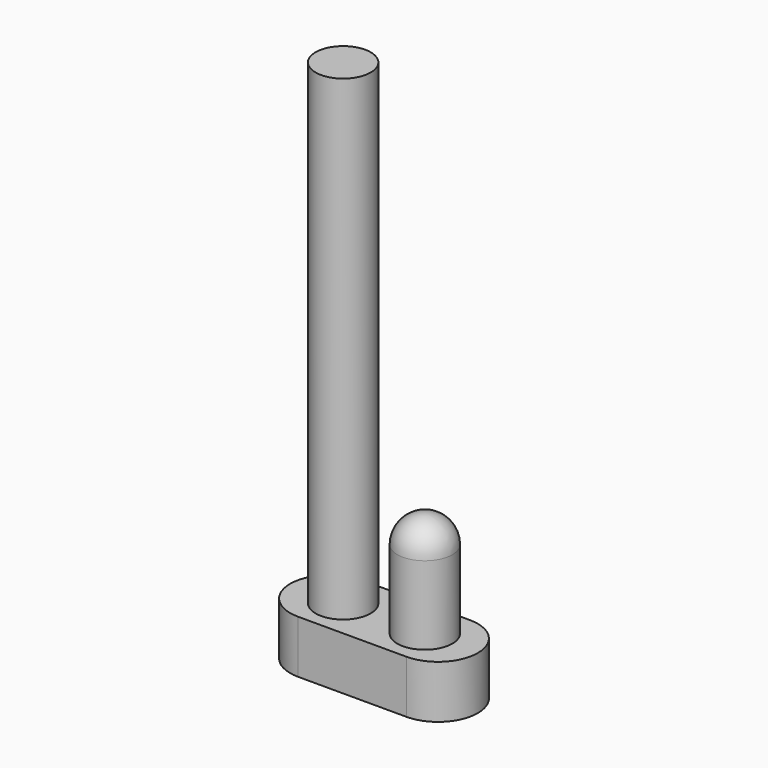
from build123d import *

# Parameters (mm, degrees)
F1_DEPTH = 63.5
F0_R     = 3.302
F2_DEPTH = 19.05
F3_DEPTH = 5.08
F4_DEPTH = 1.27
F5_R     = 3.302
F6_R     = 1.27
F7_DEPTH = 2.54


with BuildPart() as f1:
    # F0 (on Top) → F1 (new body)
    with BuildSketch(Plane.XY):
        with BuildLine():
            ThreePointArc((-3.302, 0), (0, -3.302), (3.302, 0))
            ThreePointArc((3.302, 0), (0, 3.302), (-3.302, 0))
        make_face()
    extrude(amount=F1_DEPTH)



with BuildPart() as f2:
    # F0 (on Top) → F2 (new body)
    with BuildSketch(Plane.XY):
        with Locations((9.8069049418, 0)):
            Circle(F0_R)
    extrude(amount=F2_DEPTH)


with BuildPart() as f1_1:
    add(f1.part)

    add(f2.part)  # F3 merges F2
    # F0 (on Top) → F3 (join)
    with BuildSketch(Plane.XY):
        with BuildLine():
            Line((11.3944049418, 4.7625), (-1.5875, 4.7625))
            ThreePointArc((-1.5875, 4.7625), (-6.35, 0), (-1.5875, -4.7625))
            Line((-1.5875, -4.7625), (11.3944049418, -4.7625))
            ThreePointArc((11.3944049418, -4.7625), (16.1569049418, 0), (11.3944049418, 4.7625))
        make_face()
        with BuildLine():
            ThreePointArc((-3.302, 0), (0, 3.302), (3.302, 0))
            ThreePointArc((3.302, 0), (0, -3.302), (-3.302, 0))
        make_face(mode=Mode.SUBTRACT)
        with Locations((9.8069049418, 0)):
            Circle(F0_R, mode=Mode.SUBTRACT)
    extrude(amount=F3_DEPTH)

    # F4 (add): a face of the model
    f4_faces = [f1_1.faces().sort_by_distance(p)[0] for p in [
        (4.9034524709, 0, 5.08),
    ]]
    extrude(f4_faces, amount=F4_DEPTH)

    # F5
    f5_edges = [f1_1.edges().sort_by_distance(p)[0] for p in [
        (6.504905, 0, 19.05),
    ]]
    fillet(f5_edges, radius=F5_R)

    # F6 (on face) → F7 (cut)
    with BuildSketch(Plane.XY):
        Circle(F6_R)
        with Locations((9.7663812339, 0)):
            Circle(F6_R)
    extrude(amount=F7_DEPTH, mode=Mode.SUBTRACT)


solid = f1_1.part
